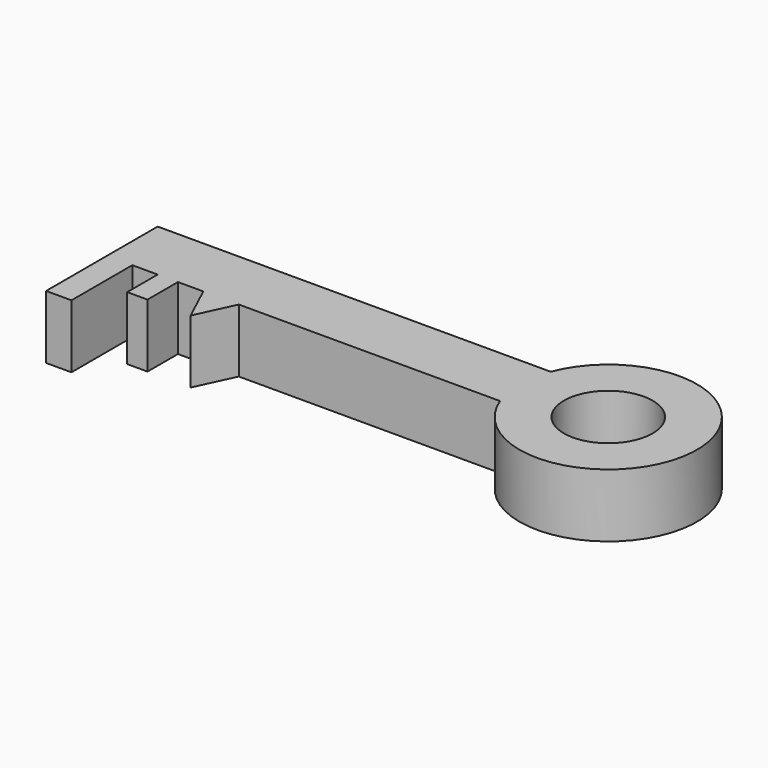
from build123d import *

# Parameters (mm, degrees)
F0_W     = 10
F0_H     = 30
F0_W_2   = 8
F0_H_2   = 15
F0_R     = 17.5
F1_DEPTH = 25


# Not quite as in the source:
# - a feature of the source that left no trace in its solid (it failed there, or was rolled back) is left out


with BuildPart() as f1:
    # F0 (on Top) → F1 (new body)
    with BuildSketch(Plane.XY):
        with Locations((-62.4986458628, -23.6081185268)):
            Rectangle(F0_W, F0_H)
        with Locations((-43.4986458628, -16.1081185268)):
            Rectangle(F0_W_2, F0_H_2)
        Polygon((87.5013541372, 16.3918814732), (-67.4986458628, 16.3918814732), (-67.4986458628, -8.6081185268), (-57.4986458628, -8.6081185268), (-47.4986458628, -8.6081185268), (-39.4986458628, -8.6081185268), (-29.4986458628, -8.6081185268), (-15.4986458628, -8.6081185268), (87.5013541372, -8.6081185268), align=None)
        Polygon((-22.4986458628, -23.6081185268), (-15.4986458628, -8.6081185268), (-29.4986458628, -8.6081185268), align=None)
        with BuildLine():
            ThreePointArc((87.5013541372, -8.6081185268), (155.1930962138, 3.8918814732), (87.5013541372, 16.3918814732))
            Line((87.5013541372, 16.3918814732), (87.5013541372, -8.6081185268))
        make_face()
        with Locations((120.1930962138, 3.8918814732)):
            Circle(F0_R, mode=Mode.SUBTRACT)
    extrude(amount=F1_DEPTH)


solid = f1.part
